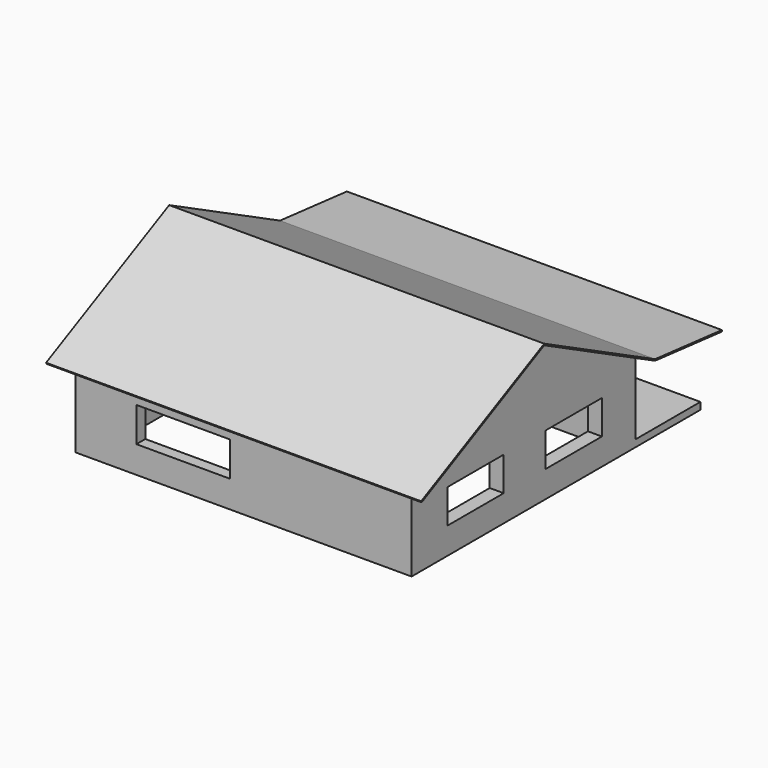
from build123d import *

# Parameters (mm, degrees)
F1_DEPTH  = 12000
F2_W      = 5000
F2_H      = 2900
F3_DEPTH  = 250
F5_DEPTH  = 700
F7_DEPTH  = 700
F8_W      = 11000
F8_H      = 9100
F9_DEPTH  = 2950
F10_W     = 2520.1079845428
F10_H     = 1213.0370140076
F11_DEPTH = 12000
F12_W     = 3353.8951873779
F12_H     = 1235.2151870728
F13_DEPTH = 10000
F14_W     = 1500.7996559143
F14_H     = 1951.2898921967
F15_DEPTH = 500


with BuildPart() as f1:
    # F0 (on Right) → F1 (new body)
    with BuildSketch(Plane.YZ):
        Polygon((-5048.6702581479, 2944.2056650102), (-5048.6702581479, 0), (4951.3297418521, 0), (7851.3297418521, 0), (7851.3297418521, 250), (4951.3297418521, 250), (4951.3297418521, 2949.7544143235), (7931.7291322167, 2653.9949799284), (7936.6666223066, 2703.7505946027), (4951.3297418521, 3000), (0, 5500), (-5048.6702581479, 3000), (-5496.7444220318, 2778.1226833141), (-5474.5566903632, 2733.3152669257), align=None)
    extrude(amount=F1_DEPTH)

    # F2 (on face) → F3 (cut)
    with BuildSketch(Plane(origin=(0, 0, 0), x_dir=(1, 0, 0), z_dir=(0, 0, -1))):
        with Locations((2500, -6401.3297418521)):
            Rectangle(F2_W, F2_H)
    extrude(amount=-F3_DEPTH, mode=Mode.SUBTRACT)

    # F4 (on face) → F5 (join)
    with BuildSketch(Plane(origin=(0, 0, 0), x_dir=(0, -1, 0), z_dir=(-1, 0, 0))):
        Polygon((5474.5566903632, 2733.3152669257), (5496.7444220318, 2778.1226833141), (0, 5500), (-4951.3297418521, 3000), (-7936.6666223066, 2703.7505946027), (-7931.7291322167, 2653.9949799284), (-4951.3297418521, 2949.7544143235), (0, 5449.7544143235), align=None)
    extrude(amount=F5_DEPTH)

    # F6 (on face) → F7 (join)
    with BuildSketch(Plane.YZ.offset(12000)):
        Polygon((-5496.7444220318, 2778.1226833141), (-5474.5566903632, 2733.3152669257), (0, 5449.7544143235), (4951.3297418521, 2949.7544143235), (7931.7291322167, 2653.9949799284), (7936.6666223066, 2703.7505946027), (4951.3297418521, 3000), (0, 5500), align=None)
    extrude(amount=F7_DEPTH)

    # F8 (on face) → F9 (cut)
    with BuildSketch(Plane(origin=(0, 0, 0), x_dir=(1, 0, 0), z_dir=(0, 0, -1))):
        with Locations((6000, 98.6702581479)):
            Rectangle(F8_W, F8_H)
    extrude(amount=-F9_DEPTH, mode=Mode.SUBTRACT)

    # F10 (on face) → F11 (cut)
    with BuildSketch(Plane(origin=(0, 0, 0), x_dir=(0, -1, 0), z_dir=(-1, 0, 0))):
        with Locations((-2193.2116746902, 1555.8831691742)):
            Rectangle(F10_W, F10_H)
        with Locations((2193.2116746902, 1555.8831691742)):
            Rectangle(F10_W, F10_H)
    extrude(amount=-F11_DEPTH, mode=Mode.SUBTRACT)

    # F12 (on face) → F13 (cut)
    with BuildSketch(Plane.XZ.offset(5048.6702581479)):
        with Locations((3844.5086479187, 1583.6279392242)):
            Rectangle(F12_W, F12_H)
    extrude(amount=-F13_DEPTH, mode=Mode.SUBTRACT)

    # F14 (on face) → F15 (cut)
    with BuildSketch(Plane(origin=(0, 4951.3297418521, 0), x_dir=(-1, 0, 0), z_dir=(0, 1, 0))):
        with Locations((-8677.9897212982, 1225.6449460983)):
            Rectangle(F14_W, F14_H)
    extrude(amount=-F15_DEPTH, mode=Mode.SUBTRACT)


solid = f1.part
